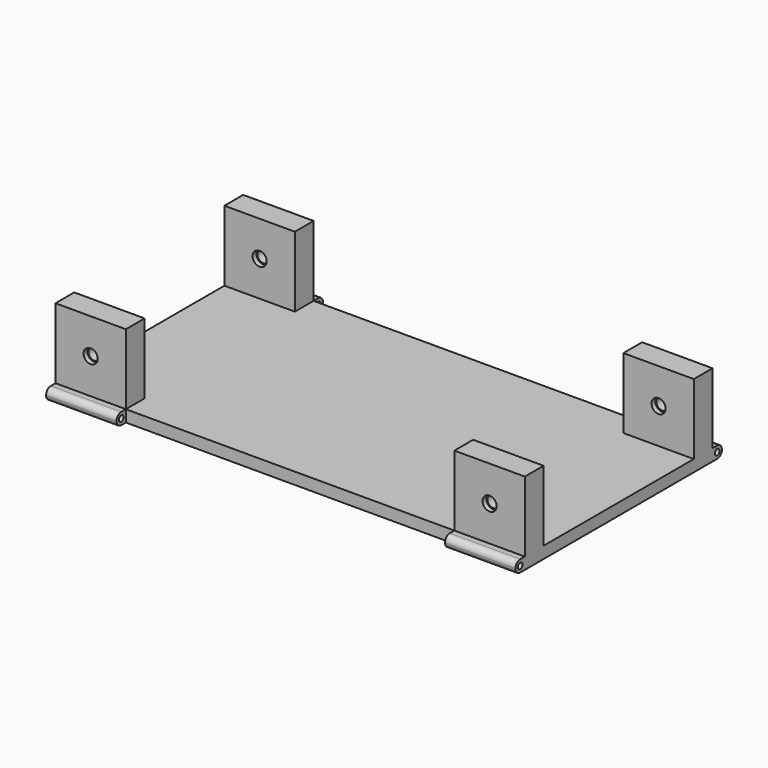
from build123d import *

# Parameters (mm, degrees)
F0_W          = 200
F0_H          = 100
F1_DEPTH      = 5
F2_W          = 30
F2_H          = 10
F3_DEPTH      = 30
F4_R          = 2.5
F5_DEPTH      = 100.001
F6_R          = 3
F6_R_2        = 2.5
F7_DEPTH      = 2
F7_DEPTH_BACK = 25
F8_R          = 3
F8_R_2        = 2.5
F9_DEPTH      = 2
F10_R         = 3
F10_R_2       = 2.5
F11_DEPTH     = 2
F12_R         = 3
F12_R_2       = 2.5
F13_DEPTH     = 2
F14_R         = 3
F14_R_2       = 2.5
F15_DEPTH     = 2
F16_R         = 3
F16_R_2       = 2.5
F17_DEPTH     = 2
F18_W         = 30
F18_H         = 5
F19_DEPTH     = 5
F20_R         = 1.25
F21_DEPTH     = 200.001
F22_R         = 2.49999
F23_W         = 30
F23_H         = 5
F24_DEPTH     = 5
F25_R         = 1.25
F26_DEPTH     = 200.001
F27_R         = 2.49999


# Not quite as in the source:
# - a fillet or chamfer is up to 0.001 mm smaller than in the source, because OpenCascade refuses the exact size


with BuildPart() as f1:
    # F0 (on Top) → F1 (new body)
    with BuildSketch(Plane.XY):
        with Locations((3.7896726225, 0)):
            Rectangle(F0_W, F0_H)
    extrude(amount=F1_DEPTH)

    # F2 (on face) → F3 (join)
    with BuildSketch(Plane.XY.offset(5)):
        with Locations((-81.2103273775, 45)):
            Rectangle(F2_W, F2_H)
        with Locations((88.7896726225, 45)):
            Rectangle(F2_W, F2_H)
        with Locations((-81.2103273775, -45)):
            Rectangle(F2_W, F2_H)
        with Locations((88.7896726225, -45)):
            Rectangle(F2_W, F2_H)
    extrude(amount=F3_DEPTH)

    # F4 (on face) → F5 (cut, through all)
    with BuildSketch(Plane.XZ.offset(50)):
        with Locations((88.7896726225, 20)):
            Circle(F4_R)
        with Locations((-81.2103273775, 20)):
            Circle(F4_R)
    extrude(amount=-F5_DEPTH, mode=Mode.SUBTRACT)

    # F6 (on face) → F7 (cut, two sides)
    with BuildSketch(Plane.XZ.offset(50)) as f7_sk:
        with Locations((88.7896726225, 20)):
            Circle(F6_R)
        with Locations((88.7896726225, 20)):
            Circle(F6_R_2, mode=Mode.SUBTRACT)
        with Locations((-81.2103273775, 20)):
            Circle(F6_R)
        with Locations((-81.2103273775, 20)):
            Circle(F6_R_2, mode=Mode.SUBTRACT)
    extrude(amount=-F7_DEPTH, mode=Mode.SUBTRACT)
    extrude(f7_sk.sketch, amount=F7_DEPTH_BACK, mode=Mode.SUBTRACT)

    # F8 (on face) → F9 (cut)
    with BuildSketch(Plane.XZ.offset(-40)):
        with Locations((-81.2103273775, 20)):
            Circle(F8_R)
        with Locations((-81.2103273775, 20)):
            Circle(F8_R_2, mode=Mode.SUBTRACT)
    extrude(amount=-F9_DEPTH, mode=Mode.SUBTRACT)

    # F10 (on face) → F11 (cut)
    with BuildSketch(Plane.XZ.offset(-40)):
        with Locations((88.7896726225, 20)):
            Circle(F10_R)
        with Locations((88.7896726225, 20)):
            Circle(F10_R_2, mode=Mode.SUBTRACT)
    extrude(amount=-F11_DEPTH, mode=Mode.SUBTRACT)

    # F12 (on face) → F13 (cut)
    with BuildSketch(Plane(origin=(0, 50, 0), x_dir=(-1, 0, 0), z_dir=(0, 1, 0))):
        with Locations((81.2103273775, 20)):
            Circle(F12_R)
        with Locations((81.2103273775, 20)):
            Circle(F12_R_2, mode=Mode.SUBTRACT)
        with Locations((-88.7896726225, 20)):
            Circle(F12_R)
        with Locations((-88.7896726225, 20)):
            Circle(F12_R_2, mode=Mode.SUBTRACT)
    extrude(amount=-F13_DEPTH, mode=Mode.SUBTRACT)

    # F14 (on face) → F15 (cut)
    with BuildSketch(Plane(origin=(0, -40, 0), x_dir=(-1, 0, 0), z_dir=(0, 1, 0))):
        with Locations((81.2103273775, 20)):
            Circle(F14_R)
        with Locations((81.2103273775, 20)):
            Circle(F14_R_2, mode=Mode.SUBTRACT)
        with Locations((81.2103273775, 20)):
            Circle(F14_R_2)
    extrude(amount=-F15_DEPTH, mode=Mode.SUBTRACT)

    # F16 (on face) → F17 (cut)
    with BuildSketch(Plane(origin=(0, -40, 0), x_dir=(-1, 0, 0), z_dir=(0, 1, 0))):
        with Locations((-88.7896726225, 20)):
            Circle(F16_R)
        with Locations((-88.7896726225, 20)):
            Circle(F16_R_2, mode=Mode.SUBTRACT)
    extrude(amount=-F17_DEPTH, mode=Mode.SUBTRACT)

    # F18 (on face) → F19 (join)
    with BuildSketch(Plane.XZ.offset(50)):
        with Locations((-81.2103273775, 2.5)):
            Rectangle(F18_W, F18_H)
        with Locations((88.7896726225, 2.5)):
            Rectangle(F18_W, F18_H)
    extrude(amount=F19_DEPTH)

    # F20 (on face) → F21 (cut, through all)
    with BuildSketch(Plane(origin=(-96.2103273775, 0, 0), x_dir=(0, -1, 0), z_dir=(-1, 0, 0))):
        with Locations((52.5, 2.5)):
            Circle(F20_R)
    extrude(amount=-F21_DEPTH, mode=Mode.SUBTRACT)

    # F22 (radius 2.5 in the source; OpenCascade refuses exactly that, so slightly less here)
    f22_edges = [f1.edges().sort_by_distance(p)[0] for p in [
        (-81.210327, -55, 5),
        (-81.210327, -55, 0),
        (88.789673, -55, 5),
        (88.789673, -55, 0),
    ]]
    fillet(f22_edges, radius=F22_R)

    # F23 (on face) → F24 (join)
    with BuildSketch(Plane(origin=(0, 50, 0), x_dir=(-1, 0, 0), z_dir=(0, 1, 0))):
        with Locations((-88.7896726225, 2.5)):
            Rectangle(F23_W, F23_H)
        with Locations((81.2103273775, 2.5)):
            Rectangle(F23_W, F23_H)
    extrude(amount=F24_DEPTH)

    # F25 (on face) → F26 (cut, through all)
    with BuildSketch(Plane(origin=(-96.2103273775, 0, 0), x_dir=(0, -1, 0), z_dir=(-1, 0, 0))):
        with Locations((-52.5, 2.5)):
            Circle(F25_R)
    extrude(amount=-F26_DEPTH, mode=Mode.SUBTRACT)

    # F27 (radius 2.5 in the source; OpenCascade refuses exactly that, so slightly less here)
    f27_edges = [f1.edges().sort_by_distance(p)[0] for p in [
        (88.789673, 55, 5),
        (88.789673, 55, 0),
        (-81.210327, 55, 0),
        (-81.210327, 55, 5),
    ]]
    fillet(f27_edges, radius=F27_R)


solid = f1.part
